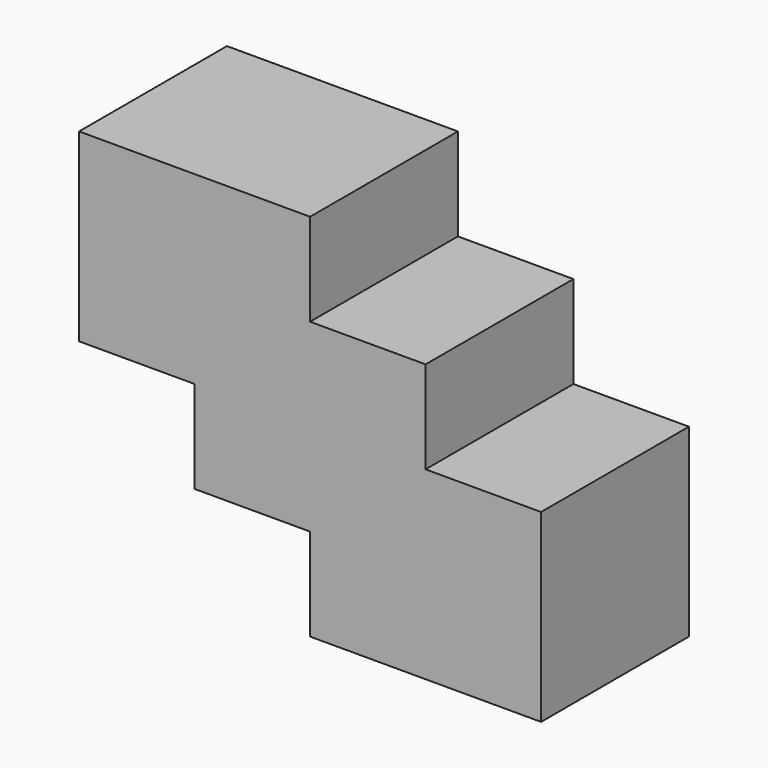
from build123d import *

# Parameters (mm, degrees)
F0_W     = 37.5
F0_H     = 30
F1_DEPTH = 60


with BuildPart() as f1:
    # F0 (on Front) → F1 (new body)
    with BuildSketch(Plane.XZ):
        with Locations((-18.75, -15)):
            Rectangle(F0_W, F0_H)
        with Locations((-18.75, 15)):
            Rectangle(F0_W, F0_H)
        with Locations((18.75, 15)):
            Rectangle(F0_W, F0_H)
        with Locations((18.75, -15)):
            Rectangle(F0_W, F0_H)
        Polygon((-75, 0), (-37.5, 0), (-37.5, 30), (0, 30), (0, 60), (-75, 60), align=None)
        Polygon((75, 0), (37.5, 0), (37.5, -30), (0, -30), (0, -60), (75, -60), align=None)
    extrude(amount=F1_DEPTH)


solid = f1.part
